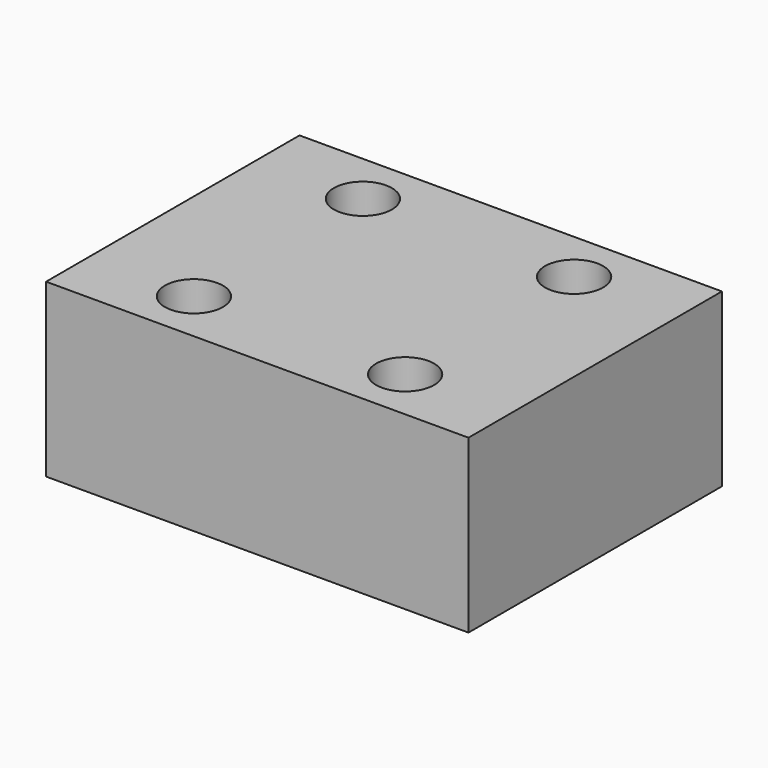
from build123d import *

# Parameters (mm, degrees)
F0_W     = 32
F0_H     = 24
F1_DEPTH = 13
F4_D     = 4.4


# Not quite as in the source:
# - a feature names something its author has since deleted; it is built from what else it names


with BuildPart() as f1:
    # F0 (on Top) → F1 (new body)
    with BuildSketch(Plane.XY):
        with Locations((0, -0.5)):
            Rectangle(F0_W, F0_H)
    extrude(amount=F1_DEPTH)

    # F4 (through all)
    with Locations(Plane.XY.offset(13)):
        with Locations((-8, 7.5), (8, 7.5), (8, -8.5), (-8, -8.5)):
            Hole(F4_D / 2)


solid = f1.part
